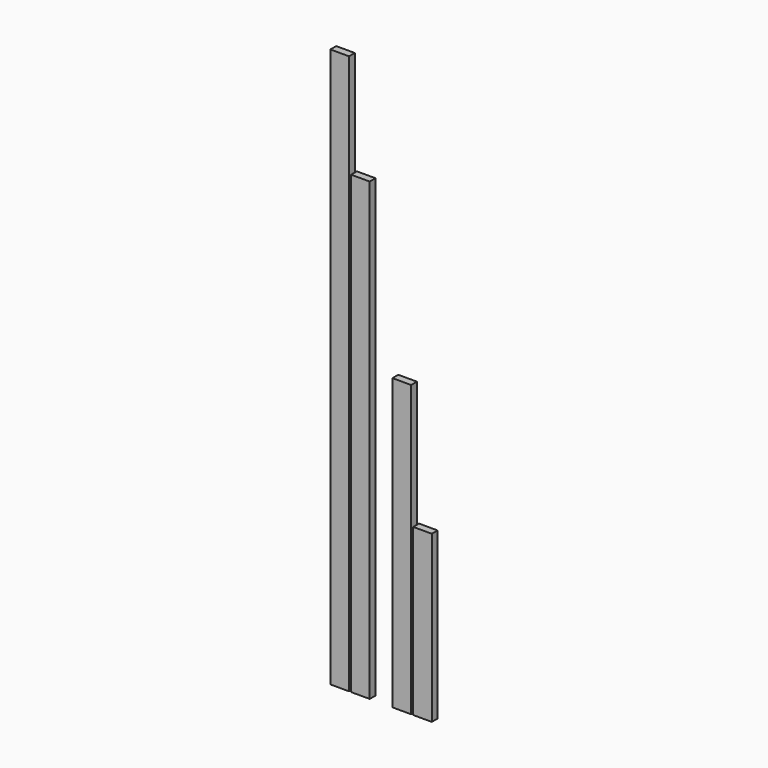
from build123d import *

# Parameters (mm, degrees)
F0_W     = 70
F0_H     = 35
F1_DEPTH = 2700
F2_DEPTH = 2200
F3_DEPTH = 1400
F4_DEPTH = 800


# Not quite as in the source:
# - a pattern or mirror of a feature is missing from the dataset's text; its kind, count and spacing are read off the source's solid


with BuildPart() as f1:
    # F0 (on Top) → F1 (new body)
    with BuildSketch(Plane.XY):
        with Locations((35, 17.5)):
            Rectangle(F0_W, F0_H)
    extrude(amount=F1_DEPTH)

    # F1_copies: F1 across plane


with BuildPart() as f1_1:
    add(f1.part)
    add(f1.part.mirror(Plane(origin=(45, 0, 0), x_dir=(0, 0, 1), z_dir=(1, 0, 0))))


with BuildPart() as f2:
    # F0 (on Top) → F2 (new body)
    with BuildSketch(Plane.XY):
        with Locations((135, 17.5)):
            Rectangle(F0_W, F0_H)
    extrude(amount=F2_DEPTH)

    # F2_copies: F2 across plane


with BuildPart() as f2_1:
    add(f2.part)
    add(f2.part.mirror(Plane(origin=(145, 0, 0), x_dir=(0, 0, 1), z_dir=(1, 0, 0))))


with BuildPart() as f3:
    # F0 (on Top) → F3 (new body)
    with BuildSketch(Plane.XY):
        with Locations((335, 17.5)):
            Rectangle(F0_W, F0_H)
    extrude(amount=F3_DEPTH)

    # F3_copies: F3 across plane


with BuildPart() as f3_1:
    add(f3.part)
    add(f3.part.mirror(Plane(origin=(345, 0, 0), x_dir=(0, 0, 1), z_dir=(1, 0, 0))))


with BuildPart() as f4:
    # F0 (on Top) → F4 (new body)
    with BuildSketch(Plane.XY):
        with Locations((435, 17.5)):
            Rectangle(F0_W, F0_H)
    extrude(amount=F4_DEPTH)

    # F4_copies: F4 across plane


with BuildPart() as f4_1:
    add(f4.part)
    add(f4.part.mirror(Plane(origin=(445, 0, 0), x_dir=(0, 0, 1), z_dir=(1, 0, 0))))


solid = Compound([f1_1.part, f2_1.part, f3_1.part, f4_1.part])
